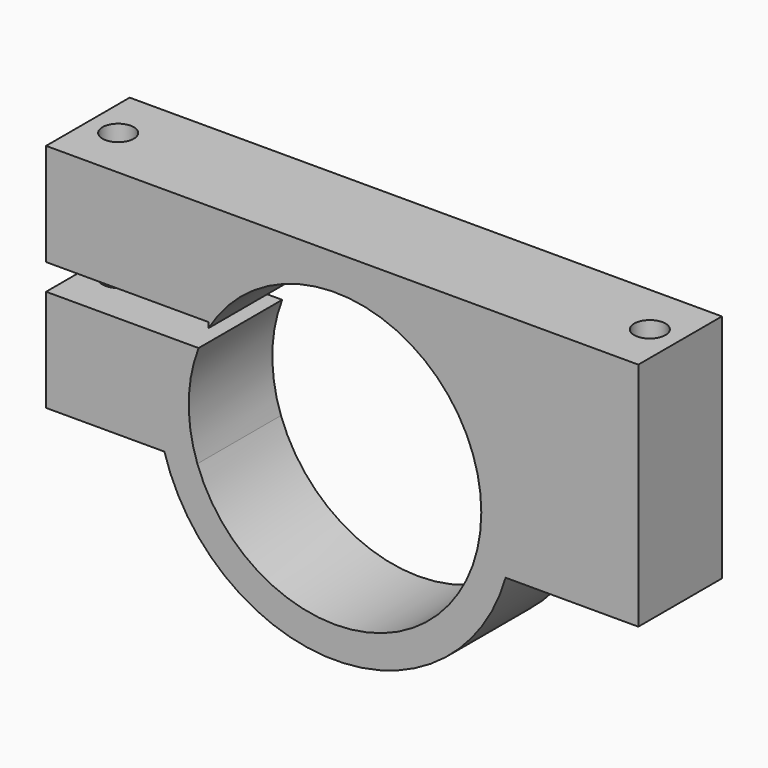
from build123d import *

# Parameters (mm, degrees)
F1_DEPTH = 12.7
F3_D     = 3.81


# Not quite as in the source:
# - a feature names something its author has since deleted; it is built from what else it names


with BuildPart() as f1:
    # F0 (on Front) → F1 (new body)
    with BuildSketch(Plane.XZ):
        with BuildLine():
            Line((-0.6058157035, 13.9202102855), (-0.6058157035, 41.9618102855))
            Line((-0.6058157035, 41.9618102855), (-2.6976561639, 41.9618102855))
            Line((-2.6976561639, 41.9618102855), (-72.5894157035, 41.9618102855))
            Line((-72.5894157035, 41.9618102855), (-72.5894157035, 29.5285102855))
            Line((-72.5894157035, 29.5285102855), (-59.4971985196, 29.5285102855))
            Line((-59.4971985196, 29.5285102855), (-56.8120155754, 29.5285102855))
            ThreePointArc((-56.8120155754, 29.5285102855), (-32.5437541307, 40.9543939264), (-15.88096278, 19.934148568))
            ThreePointArc((-15.88096278, 19.934148568), (-16.0956571498, 16.8969773161), (-16.7354703496, 13.9202102855))
            Line((-16.7354703496, 13.9202102855), (-0.6058157035, 13.9202102855))
        make_face()
        with BuildLine():
            Line((-72.5894157035, 13.9202102855), (-58.2064552105, 13.9202102855))
            ThreePointArc((-58.2064552105, 13.9202102855), (-59.0599250667, 20.1458261131), (-58.0845479883, 26.3535102855))
            Line((-58.0845479883, 26.3535102855), (-59.4971985196, 26.3535102855))
            Line((-59.4971985196, 26.3535102855), (-72.5894157035, 26.3535102855))
            Line((-72.5894157035, 26.3535102855), (-72.5894157035, 13.9202102855))
        make_face()
        with BuildLine():
            Line((-20.7389292415, 13.9202102855), (-16.7354703496, 13.9202102855))
            ThreePointArc((-16.7354703496, 13.9202102855), (-16.0956571498, 16.8969773161), (-15.88096278, 19.934148568))
            ThreePointArc((-15.88096278, 19.934148568), (-32.5437541307, 40.9543939264), (-56.8120155754, 29.5285102855))
            Line((-56.8120155754, 29.5285102855), (-52.8308911926, 29.5285102855))
            Line((-52.8308911926, 29.5285102855), (-52.8308911926, 28.8896496238))
            ThreePointArc((-52.8308911926, 28.8896496238), (-32.8325970751, 37.098470972), (-19.69096278, 19.934148568))
            ThreePointArc((-19.69096278, 19.934148568), (-19.9549136205, 16.881867152), (-20.7389292415, 13.9202102855))
        make_face()
        with BuildLine():
            ThreePointArc((-58.2064552105, 13.9202102855), (-37.47096278, -1.655851432), (-16.7354703496, 13.9202102855))
            Line((-16.7354703496, 13.9202102855), (-20.7389292415, 13.9202102855))
            ThreePointArc((-20.7389292415, 13.9202102855), (-37.47096278, 2.154148568), (-54.2029963185, 13.9202102855))
            Line((-54.2029963185, 13.9202102855), (-58.2064552105, 13.9202102855))
        make_face()
        with BuildLine():
            ThreePointArc((-58.0845479883, 26.3535102855), (-59.0599250667, 20.1458261131), (-58.2064552105, 13.9202102855))
            Line((-58.2064552105, 13.9202102855), (-54.2029963185, 13.9202102855))
            ThreePointArc((-54.2029963185, 13.9202102855), (-55.249646191, 20.1505190165), (-54.0516803501, 26.3535102855))
            Line((-54.0516803501, 26.3535102855), (-58.0845479883, 26.3535102855))
        make_face()
    extrude(amount=F1_DEPTH)

    # F3 (through all)
    with Locations(Plane(origin=(0, 0, 0), x_dir=(1, 0, 0), z_dir=(0, 0, -1))):
        with Locations((-68.9064157035, 6.35), (-4.2888157035, 6.35)):
            Hole(F3_D / 2)


solid = f1.part
